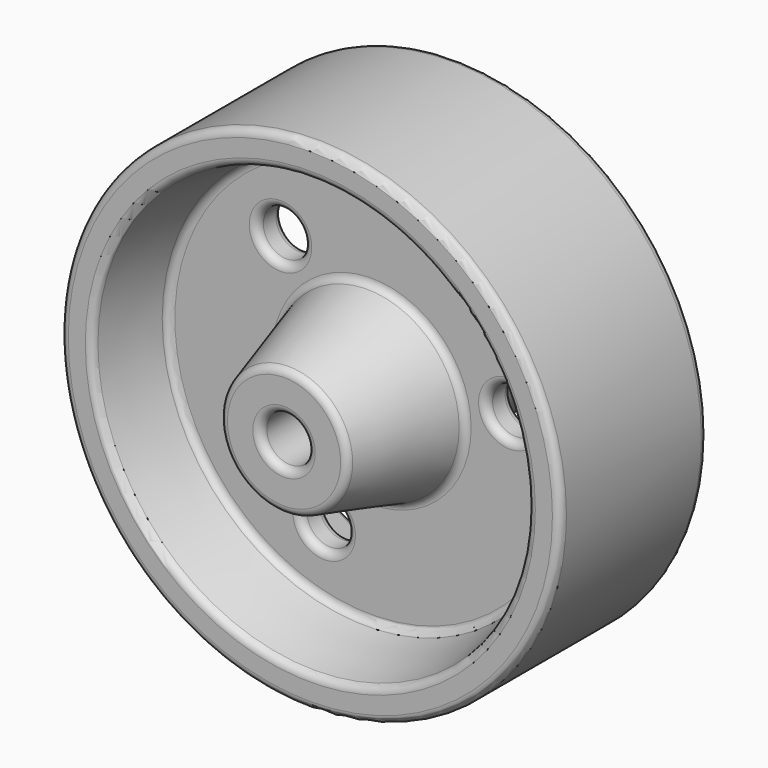
from build123d import *

# Parameters (mm, degrees)
F2_R     = 4.7625
F3_DEPTH = 50.801
F4_R     = 1.5875
F5_R     = 1.5875


# Not quite as in the source:
# - the program builds the solid bodies; features that only make, move or delete a surface that nothing else refers to are left out


with BuildPart() as f1:
    # F0 (on Top) → F1 (revolve)
    with BuildSketch(Plane.XY):
        Polygon((-17.0852003332, 29.4403855965), (-29.7852003332, 29.4403855965), (-29.7852003332, -21.3596144035), (-17.0852003332, -21.3596144035), (-10.726400651, 0.8653855965), (11.4897996668, 0.8653855965), (14.6647996668, -14.6774463356), (21.0147996668, -14.6774463356), (21.0147996668, 0.8653855965), (21.0147996668, 4.0403855965), (21.0147996668, 22.7582119405), (14.6647996668, 22.7582119405), (11.4897996668, 7.2153855965), (-10.726400651, 7.2153855965), align=None)
    revolve(axis=Axis((-29.7852003332, 4.0403855965, 0), (0, -1, 0)))

    # F2 (on face) → F3 (cut, through all)
    with BuildSketch(Plane(origin=(0, 29.4403855965, 0), x_dir=(-1, 0, 0), z_dir=(0, 1, 0))):
        with Locations((29.7852003332, 0)):
            Circle(F2_R)
        with Locations((39.3995883172, -26.9089979132)):
            Circle(F2_R)
        with Locations((48.2818821243, 21.7808031926)):
            Circle(F2_R)
        with Locations((1.6741305579, 5.1281947206)):
            Circle(F2_R)
    extrude(amount=-F3_DEPTH, mode=Mode.SUBTRACT)

    # F4
    f4_edges = [f1.edges().sort_by_distance(p)[0] for p in [
        (-25.0227, 29.440386, 0),
        (-42.4852, 29.440386, 0),
        (-48.844, 7.215386, 0),
        (-43.519382, 7.215386, 21.780803),
        (3.088369, 7.215386, 5.128195),
        (-34.637088, 7.215386, -26.908998),
        (-71.0602, 7.215386, 0),
        (-74.2352, 22.758212, 0),
        (-80.5852, 22.758212, 0),
    ]]
    fillet(f4_edges, radius=F4_R)

    # F5
    f5_edges = [f1.edges().sort_by_distance(p)[0] for p in [
        (-25.0227, -21.359614, 0),
        (-42.4852, -21.359614, 0),
        (-48.844, 0.865386, 0),
        (-43.519382, 0.865386, 21.780803),
        (3.088369, 0.865386, 5.128195),
        (-34.637088, 0.865386, -26.908998),
        (-71.0602, 0.865386, 0),
        (-74.2352, -14.677446, 0),
        (-80.5852, -14.677446, 0),
    ]]
    fillet(f5_edges, radius=F5_R)


solid = f1.part
